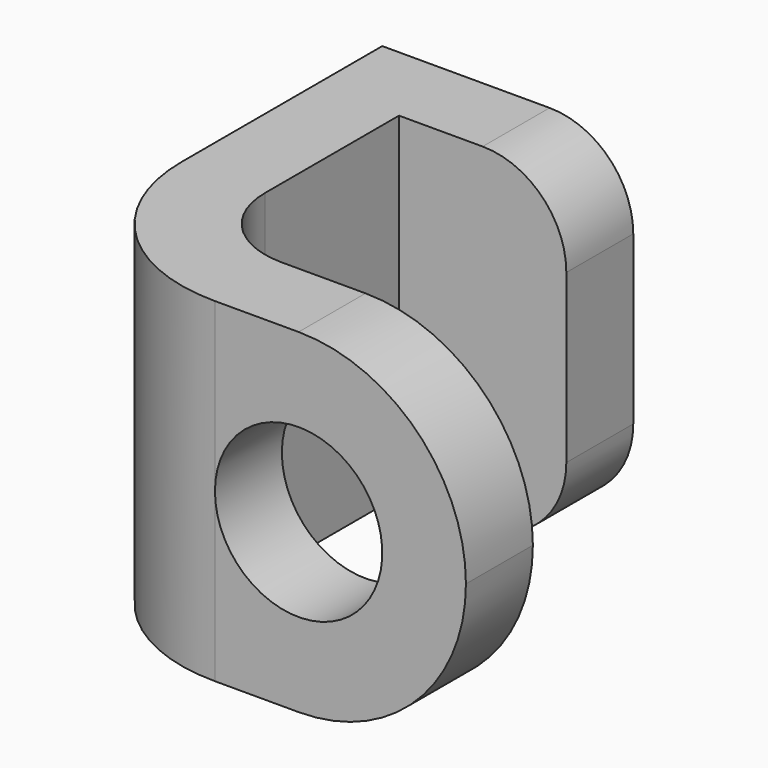
from build123d import *

# Parameters (mm, degrees)
F1_DEPTH = 20
F2_R     = 10
F3_R     = 19.99999
F4_R     = 10
F5_DEPTH = 10.001


# Not quite as in the source:
# - a fillet or chamfer is up to 0.001 mm smaller than in the source, because OpenCascade refuses the exact size


with BuildPart() as f1:
    # F0 (on Top) → F1 (new body, symmetric)
    with BuildSketch(Plane.XY):
        with BuildLine():
            ThreePointArc((10, 0), (2.9289321881, 2.9289321881), (0, 10))
            Line((0, 10), (0, 30))
            Line((0, 30), (20, 30))
            Line((20, 30), (20, 40))
            Line((20, 40), (-10, 40))
            Line((-10, 40), (-10, 10))
            ThreePointArc((-10, 10), (-4.1421356237, -4.1421356237), (10, -10))
            Line((10, -10), (40, -10))
            Line((40, -10), (40, 0))
            Line((40, 0), (10, 0))
        make_face()
    extrude(amount=F1_DEPTH, both=True)

    # F2
    f2_edges = [f1.edges().sort_by_distance(p)[0] for p in [
        (20, 35, 20),
        (20, 35, -20),
    ]]
    fillet(f2_edges, radius=F2_R)

    # F3 (radius 20 in the source; OpenCascade refuses exactly that, so slightly less here)
    f3_edges = [f1.edges().sort_by_distance(p)[0] for p in [
        (40, -5, 20),
        (40, -5, -20),
    ]]
    fillet(f3_edges, radius=F3_R)

    # F4 (on face) → F5 (cut, through all)
    with BuildSketch(Plane(origin=(0, 0, 0), x_dir=(-1, 0, 0), z_dir=(0, 1, 0))):
        with Locations((-20, 0)):
            Circle(F4_R)
    extrude(amount=-F5_DEPTH, mode=Mode.SUBTRACT)


solid = f1.part
